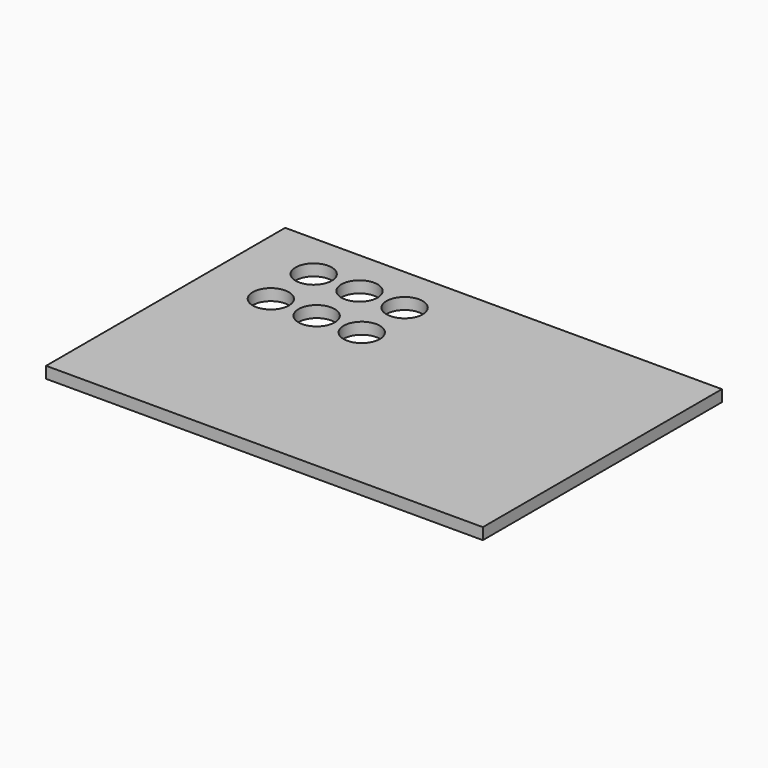
from build123d import *

# Parameters (mm, degrees)
F0_W     = 361.95
F0_H     = 247.65
F1_DEPTH = 9.525
F3_D     = 30


# Not quite as in the source:
# - a feature names something its author has since deleted; it is built from what else it names


with BuildPart() as f1:
    # F0 (on Top) → F1 (new body)
    with BuildSketch(Plane.XY):
        with Locations((-148.0553561452, 71.3610090315)):
            Rectangle(F0_W, F0_H)
    extrude(amount=-F1_DEPTH)

    # F3 (through all)
    with Locations(Plane(origin=(0, 0, -9.525), x_dir=(1, 0, 0), z_dir=(0, 0, -1))):
        with Locations((-236.1291795969, -111.6871535778), (-236.1291795969, -156.0809910297), (-198.7664848566, -111.6871535778), (-274.1136550903, -156.0809910297), (-198.7664848566, -156.0809910297), (-274.1136550903, -111.6871535778)):
            Hole(F3_D / 2)


solid = f1.part
